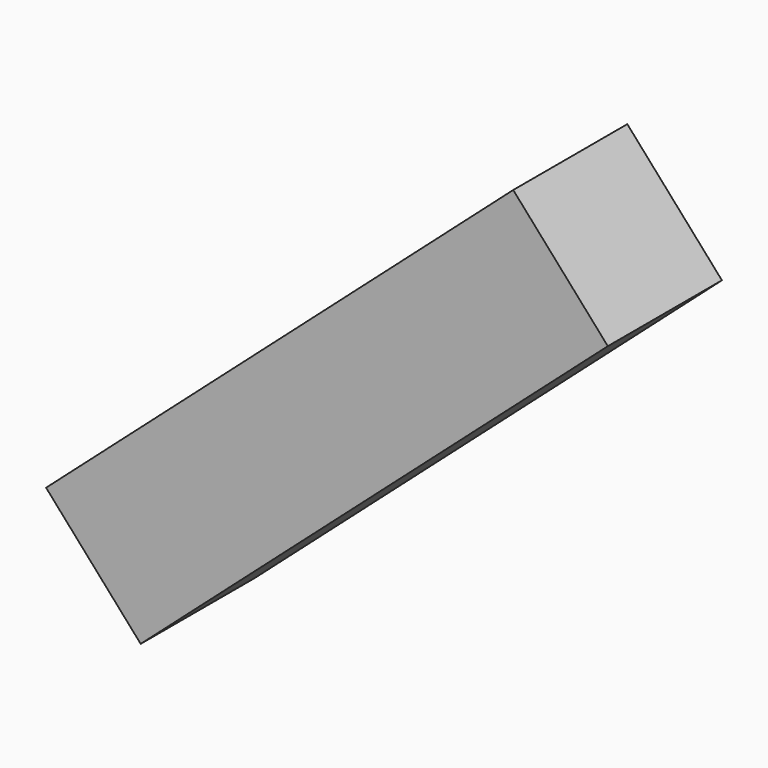
from build123d import *

# Parameters (mm, degrees)
F1_E2_W  = 111.164008953
F1_E2_H  = 25.4
F2_DEPTH = 25.4


with BuildPart() as f2:
    # F1_E2 (on explicit) → F2 (new body)
    with BuildSketch(Plane(origin=(-6.1802798882, 0, -73.7301930785), x_dir=(0.7483926191, 0, 0.6632559744), z_dir=(0.6632559744, 0, -0.7483926191))):
        with Locations((55.5820044765, 12.7)):
            Rectangle(F1_E2_W, F1_E2_H)
    extrude(amount=F2_DEPTH)


solid = f2.part
